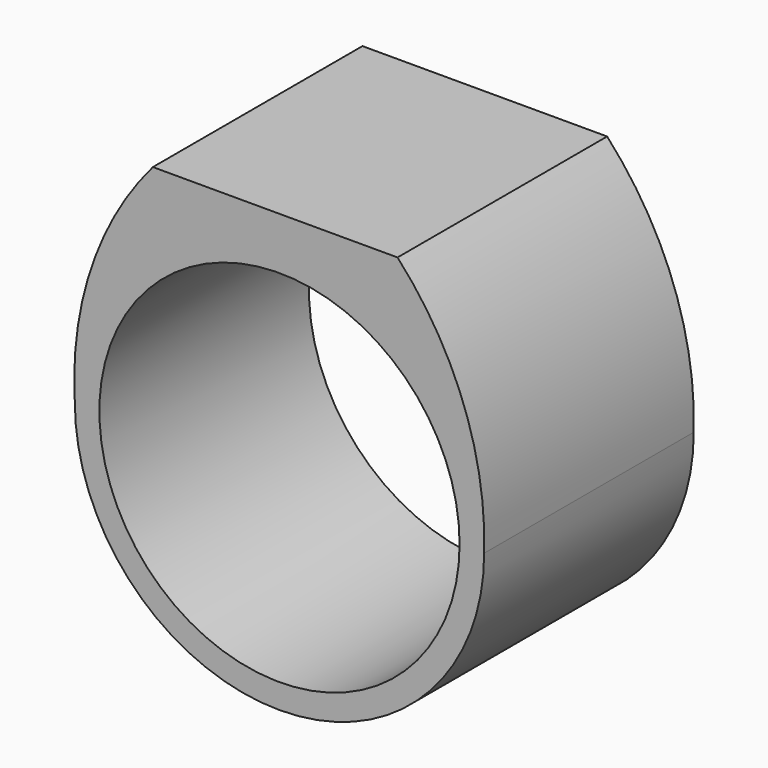
from build123d import *

# Parameters (mm, degrees)
F0_R     = 12.5
F0_R_2   = 11
F1_DEPTH = 16
F3_DEPTH = 16
F4_DEPTH = 26
F6_DEPTH = 16


# Not quite as in the source:
# - a feature of the source that left no trace in its solid (it failed there, or was rolled back) is left out
# - a feature names something its author has since deleted; it is built from what else it names


with BuildPart() as f1:
    # F0 (on Front) → F1 (new body)
    with BuildSketch(Plane.XZ):
        Circle(F0_R)
        Circle(F0_R_2, mode=Mode.SUBTRACT)
    extrude(amount=F1_DEPTH)

    # F2 (on Front) → F3 (join)
    with BuildSketch(Plane.XZ):
        with BuildLine():
            Line((7.2098509409, 14.1820398122), (-7.7328206971, 14.1820398122))
            Line((-7.7328206971, 14.1820398122), (-7.7328206971, 9.7571304068))
            ThreePointArc((-7.7328206971, 9.7571304068), (0.3692249529, -12.210413225), (7.2098509409, 10.1820398122))
            Line((7.2098509409, 10.1820398122), (7.2098509409, 14.1820398122))
        make_face()
    extrude(amount=F3_DEPTH)

    # F0 (on Front) → F4 (cut)
    with BuildSketch(Plane.XZ):
        Circle(F0_R_2)
    extrude(amount=F4_DEPTH, mode=Mode.SUBTRACT)

    # F5 (on face) → F6 (join)
    with BuildSketch(Plane.XZ.offset(16)):
        with BuildLine():
            ThreePointArc((-7.7328206971, 14.1820398122), (-11.492539371, 7.5535946754), (-12.5, 0))
            ThreePointArc((-12.5, 0), (-11.2452269589, 5.4584677926), (-7.7328206971, 9.8210734681))
            Line((-7.7328206971, 9.8210734681), (-7.7328206971, 14.1820398122))
        make_face()
        with BuildLine():
            ThreePointArc((7.2098509409, 10.2111727735), (11.0989444715, 5.7500810098), (12.5, 0))
            ThreePointArc((12.5, 0), (11.2484098162, 7.6108139553), (7.2098509409, 14.1820398122))
            Line((7.2098509409, 14.1820398122), (7.2098509409, 10.2111727735))
        make_face()
    extrude(amount=-F6_DEPTH)


solid = f1.part
